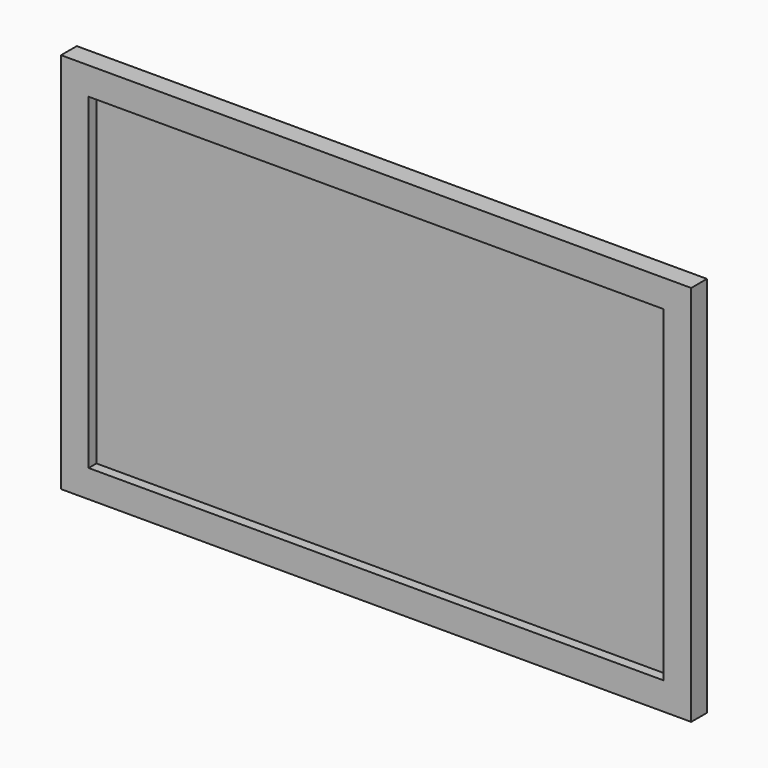
from build123d import *

# Parameters (mm, degrees)
F0_W        = 927.1
F0_H        = 527.05
F1_DEPTH    = 12.7
F2_W        = 1016
F2_H        = 615.95
F2_W_2      = 927.1
F2_H_2      = 527.05
F3_DEPTH    = 15.875
F4_W        = 965.2
F4_H        = 558.8
F5_DEPTH    = 25.4
F6_T1_DEPTH = 842.7806331425
F6_T3_DEPTH = 1249.1806331425


# Not quite as in the source:
# - a fillet or chamfer that OpenCascade refuses, or shapes differently, is made with other operations: its cross-section is extruded or revolved along the edge and cut away or added


with BuildPart() as f1:
    # F0 (on Front) → F1 (new body)
    with BuildSketch(Plane.XZ):
        Rectangle(F0_W, F0_H)
    extrude(amount=F1_DEPTH)


with BuildPart() as f3:
    # F2 (on face) → F3 (new body, symmetric)
    with BuildSketch(Plane.XZ.offset(12.7)):
        Rectangle(F2_W, F2_H)
        Rectangle(F2_W_2, F2_H_2, mode=Mode.SUBTRACT)
    extrude(amount=F3_DEPTH, both=True)

    # F4 (on face) → F5 (join)
    with BuildSketch(Plane(origin=(0, 3.175, 0), x_dir=(-1, 0, 0), z_dir=(0, 1, 0))):
        Rectangle(F4_W, F4_H)
    extrude(amount=F5_DEPTH)

    # F6: fillet of radius 76.2 on 4 edges, made by hand

    # F6_s2 → F6_t1 (cut)
    with BuildSketch(Plane.XY.offset(-421.3903165712)):
        with BuildLine():
            ThreePointArc((482.6, 3.175), (456.9123931049, 21.9357648032), (425.8038733715, 28.575))
            Line((425.8038733715, 28.575), (425.8038733715, 30.099))
            Line((425.8038733715, 30.099), (482.6, 30.099))
            Line((482.6, 30.099), (484.124, 28.575))
            ThreePointArc((484.124, 28.575), (484.124, 15.875), (483.7359225326, 4.191))
            Line((483.7359225326, 4.191), (482.6, 3.175))
        make_face()
        with BuildLine():
            ThreePointArc((-482.6, 3.175), (-456.9123931049, 21.9357648032), (-425.8038733715, 28.575))
            Line((-425.8038733715, 28.575), (-425.8038733715, 30.099))
            Line((-425.8038733715, 30.099), (-482.6, 30.099))
            Line((-482.6, 30.099), (-484.124, 28.575))
            ThreePointArc((-484.124, 28.575), (-484.124, 15.875), (-483.7359225326, 4.191))
            Line((-483.7359225326, 4.191), (-482.6, 3.175))
        make_face()
    extrude(amount=F6_T1_DEPTH, mode=Mode.SUBTRACT)

    # F6_s4 → F6_t3 (cut)
    with BuildSketch(Plane.YZ.offset(-624.5903165712)):
        with BuildLine():
            ThreePointArc((3.175, 279.4), (21.9357648032, 253.7123931049), (28.575, 222.6038733715))
            Line((28.575, 222.6038733715), (30.099, 222.6038733715))
            Line((30.099, 222.6038733715), (30.099, 279.4))
            Line((30.099, 279.4), (28.575, 280.924))
            ThreePointArc((28.575, 280.924), (15.875, 280.924), (4.191, 280.5359225326))
            Line((4.191, 280.5359225326), (3.175, 279.4))
        make_face()
        with BuildLine():
            ThreePointArc((3.175, -279.4), (21.9357648032, -253.7123931049), (28.575, -222.6038733715))
            Line((28.575, -222.6038733715), (30.099, -222.6038733715))
            Line((30.099, -222.6038733715), (30.099, -279.4))
            Line((30.099, -279.4), (28.575, -280.924))
            ThreePointArc((28.575, -280.924), (15.875, -280.924), (4.191, -280.5359225326))
            Line((4.191, -280.5359225326), (3.175, -279.4))
        make_face()
    extrude(amount=F6_T3_DEPTH, mode=Mode.SUBTRACT)


solid = Compound([f1.part, f3.part])
